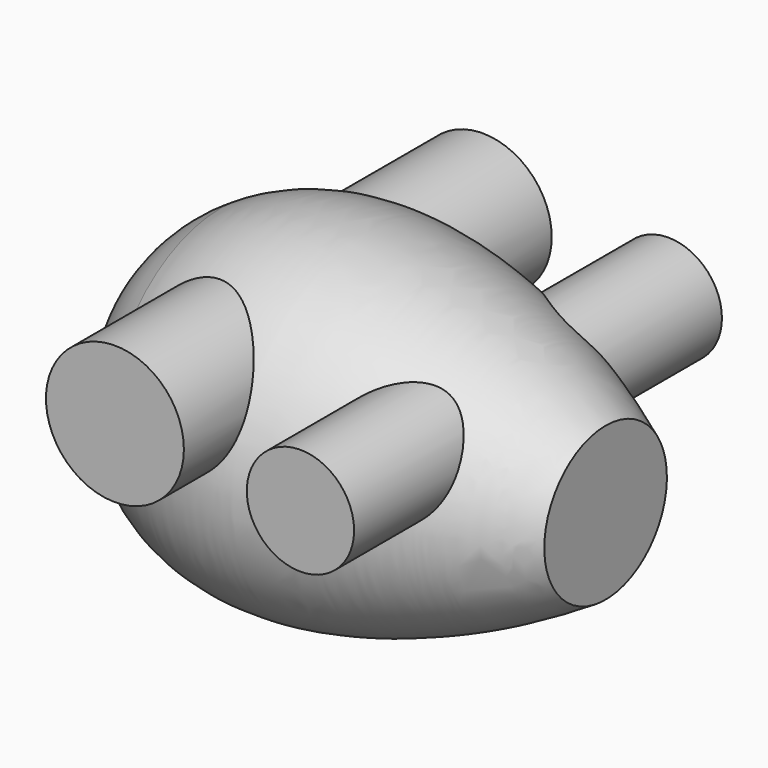
from build123d import *

# Parameters (mm, degrees)
F3_R   = 7
F3_R_2 = 9


# Not quite as in the source:
# - a pattern or mirror of a feature is missing from the dataset's text; its kind, count and spacing are read off the source's solid


with BuildPart() as f1:
    # F0 (on Front) → F1 (revolve)
    with BuildSketch(Plane.XZ):
        with BuildLine():
            Line((-61, 0), (0, 0))
            Line((0, 0), (0, 10))
            add(Edge.make_bspline(
                [(-50.25, 18.6195461814), (-37.2210499958, 26.1418139735), (-10.4841707805, 16.6390100311), (-3.3322397366, 11.9742266545), (0, 10)],
                knots=[0, 0, 0, 0, 0.6387203747, 1, 1, 1, 1], degree=3))
            ThreePointArc((-50.25, 18.6195461814), (-58.1195461814, 10.75), (-61, 0))
        make_face()
    revolve(axis=Axis((-30.5, 0, 0), (-1, 0, 0)))

    # F3 (on offset) → F4 (join, up to the next surface of F1)
    with BuildSketch(Plane.XZ.offset(30)):
        with Locations((-15.8201763071, 7.2742023454)):
            Circle(F3_R)
        with Locations((-40.0313028448, 9.3763558499)):
            Circle(F3_R_2)
    f4 = extrude(until=Until.NEXT, dir=(0, 1, 0))

    # F4_copies: F4 across plane
    add(f4.mirror(Plane.ZX))


solid = f1.part
